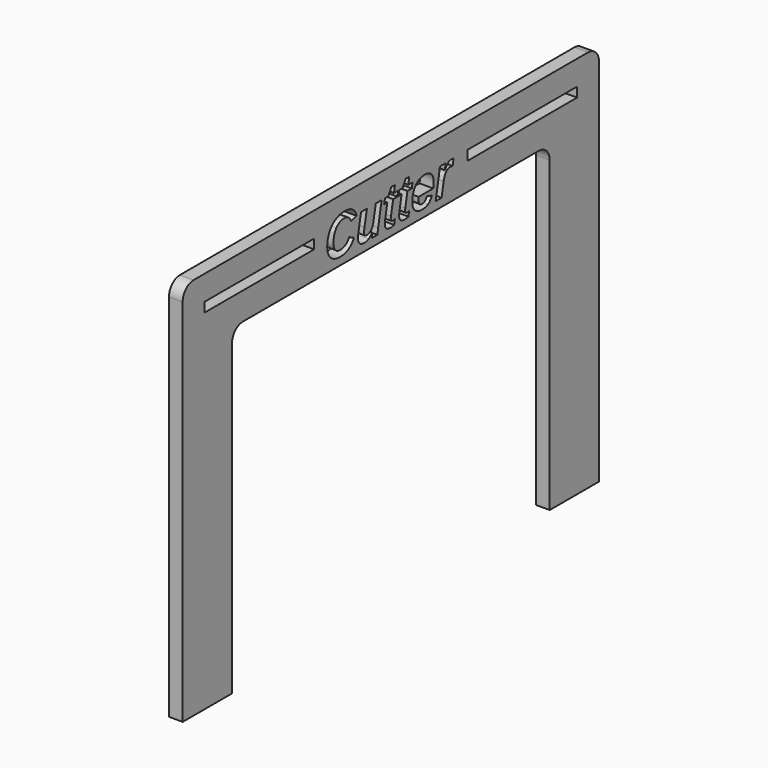
from build123d import *

# Parameters (mm, degrees)
F0_W     = 63.5
F0_H     = 4.4112131
F0_H_2   = 4.4905743218
F0_W_2   = 28.575
F0_H_3   = 149.225
F1_DEPTH = 6.35
F2_R     = 6.35


with BuildPart() as f1:
    # F0 (on Right) → F1 (new body)
    with BuildSketch(Plane.YZ):
        Polygon((-136.4888010454, 79.3362986231), (-136.4888010454, 50.7612986231), (-107.9138010454, 50.7612986231), (76.2361989546, 50.7612986231), (104.8111989546, 50.7612986231), (104.8111989546, 79.3362986231), align=None)
        with Locations((-92.0388010454, 65.6669051731)):
            Rectangle(F0_W, F0_H, mode=Mode.SUBTRACT)
        with BuildLine():
            add(Edge.make_bspline(
                [(-47.3880220701, 67.0227738236), (-49.0617207982, 64.9793044462), (-49.0617207982, 61.4645371172)],
                knots=[0, 0, 0, 1, 1, 1], degree=2))
            add(Edge.make_bspline(
                [(-49.0617207982, 61.4645371172), (-49.0617207982, 59.3587905779), (-48.0205244964, 58.2086092427)],
                knots=[0, 0, 0, 1, 1, 1], degree=2))
            add(Edge.make_bspline(
                [(-48.0205244964, 58.2086092427), (-46.9793281946, 57.0584279074), (-45.0487361733, 57.0584279074)],
                knots=[0, 0, 0, 1, 1, 1], degree=2))
            add(Edge.make_bspline(
                [(-45.0487361733, 57.0584279074), (-41.8103237506, 57.0584279074), (-39.9614705044, 60.1995322646)],
                knots=[0, 0, 0, 1, 1, 1], degree=2))
            Line((-39.9614705044, 60.1995322646), (-37.2018137644, 58.7749421844))
            add(Edge.make_bspline(
                [(-37.2018137644, 58.7749421844), (-39.7551774054, 54.2481709733), (-45.290060176, 54.2481709733)],
                knots=[0, 0, 0, 1, 1, 1], degree=2))
            add(Edge.make_bspline(
                [(-45.290060176, 54.2481709733), (-47.6137767822, 54.2481709733), (-49.2991524782, 55.1258897249)],
                knots=[0, 0, 0, 1, 1, 1], degree=2))
            add(Edge.make_bspline(
                [(-49.2991524782, 55.1258897249), (-50.9845281742, 56.0036084765), (-51.8525161192, 57.6267070105)],
                knots=[0, 0, 0, 1, 1, 1], degree=2))
            add(Edge.make_bspline(
                [(-51.8525161192, 57.6267070105), (-52.7205040642, 59.2498055445), (-52.7205040642, 61.4139369231)],
                knots=[0, 0, 0, 1, 1, 1], degree=2))
            add(Edge.make_bspline(
                [(-52.7205040642, 61.4139369231), (-52.7205040642, 64.4810871504), (-51.4438222437, 66.894327177)],
                knots=[0, 0, 0, 1, 1, 1], degree=2))
            add(Edge.make_bspline(
                [(-51.4438222437, 66.894327177), (-50.1671404232, 69.3075672035), (-47.874562398, 70.5978721532)],
                knots=[0, 0, 0, 1, 1, 1], degree=2))
            add(Edge.make_bspline(
                [(-47.874562398, 70.5978721532), (-45.5819843728, 71.8881771029), (-42.6627424051, 71.8881771029)],
                knots=[0, 0, 0, 1, 1, 1], degree=2))
            add(Edge.make_bspline(
                [(-42.6627424051, 71.8881771029), (-39.8641624389, 71.8881771029), (-38.0698017094, 70.6893417349)],
                knots=[0, 0, 0, 1, 1, 1], degree=2))
            add(Edge.make_bspline(
                [(-38.0698017094, 70.6893417349), (-36.27544098, 69.4905063669), (-35.6565616829, 67.1200818892)],
                knots=[0, 0, 0, 1, 1, 1], degree=2))
            Line((-35.6565616829, 67.1200818892), (-38.9883898486, 66.2559862667))
            add(Edge.make_bspline(
                [(-38.9883898486, 66.2559862667), (-39.3425912073, 67.556022023), (-40.3390257989, 68.3111326119)],
                knots=[0, 0, 0, 1, 1, 1], degree=2))
            add(Edge.make_bspline(
                [(-40.3390257989, 68.3111326119), (-41.3354603905, 69.0662432009), (-42.7717274386, 69.0662432009)],
                knots=[0, 0, 0, 1, 1, 1], degree=2))
            add(Edge.make_bspline(
                [(-42.7717274386, 69.0662432009), (-45.714323342, 69.0662432009), (-47.3880220701, 67.0227738236)],
                knots=[0, 0, 0, 1, 1, 1], degree=2))
        make_face(mode=Mode.SUBTRACT)
        with BuildLine():
            Line((-33.1148750097, 67.6533300886), (-29.7207696821, 67.6533300886))
            Line((-29.7207696821, 67.6533300886), (-31.1570367301, 60.4175023315))
            add(Edge.make_bspline(
                [(-31.1570367301, 60.4175023315), (-31.4723148626, 58.9228504441), (-31.4723148626, 58.4090638578)],
                knots=[0, 0, 0, 1, 1, 1], degree=2))
            add(Edge.make_bspline(
                [(-31.4723148626, 58.4090638578), (-31.4723148626, 56.8404578405), (-29.6234616165, 56.8404578405)],
                knots=[0, 0, 0, 1, 1, 1], degree=2))
            add(Edge.make_bspline(
                [(-29.6234616165, 56.8404578405), (-28.3934876674, 56.8404578405), (-27.354237527, 57.8252154643)],
                knots=[0, 0, 0, 1, 1, 1], degree=2))
            add(Edge.make_bspline(
                [(-27.354237527, 57.8252154643), (-26.3149873865, 58.809973088), (-26.0347401576, 60.2851633623)],
                knots=[0, 0, 0, 1, 1, 1], degree=2))
            Line((-26.0347401576, 60.2851633623), (-24.5984731095, 67.6533300886))
            Line((-24.5984731095, 67.6533300886), (-21.1693368783, 67.6533300886))
            Line((-21.1693368783, 67.6533300886), (-23.1894523198, 57.3036442327))
            add(Edge.make_bspline(
                [(-23.1894523198, 57.3036442327), (-23.384068451, 56.3422405447), (-23.652638712, 54.4933872986)],
                knots=[0, 0, 0, 1, 1, 1], degree=2))
            Line((-23.652638712, 54.4933872986), (-26.9105127479, 54.4933872986))
            add(Edge.make_bspline(
                [(-26.9105127479, 54.4933872986), (-26.9105127479, 54.602372332), (-26.7956892305, 55.5151219872)],
                knots=[0, 0, 0, 1, 1, 1], degree=2))
            add(Edge.make_bspline(
                [(-26.7956892305, 55.5151219872), (-26.6808657131, 56.4278716424), (-26.6185885511, 56.7431497749)],
                knots=[0, 0, 0, 1, 1, 1], degree=2))
            Line((-26.6185885511, 56.7431497749), (-26.6536194547, 56.7431497749))
            add(Edge.make_bspline(
                [(-26.6536194547, 56.7431497749), (-27.5799922391, 55.4431140187), (-28.6815195416, 54.8534271412)],
                knots=[0, 0, 0, 1, 1, 1], degree=2))
            add(Edge.make_bspline(
                [(-28.6815195416, 54.8534271412), (-29.783046844, 54.2637402638), (-31.1920676337, 54.2637402638)],
                knots=[0, 0, 0, 1, 1, 1], degree=2))
            add(Edge.make_bspline(
                [(-31.1920676337, 54.2637402638), (-33.0409208799, 54.2637402638), (-33.9770244708, 55.1511898219)],
                knots=[0, 0, 0, 1, 1, 1], degree=2))
            add(Edge.make_bspline(
                [(-33.9770244708, 55.1511898219), (-34.9131280618, 56.0386393801), (-34.9131280618, 57.7162304308)],
                knots=[0, 0, 0, 1, 1, 1], degree=2))
            add(Edge.make_bspline(
                [(-34.9131280618, 57.7162304308), (-34.9131280618, 58.0198315954), (-34.8294431254, 58.6951495706)],
                knots=[0, 0, 0, 1, 1, 1], degree=2))
            add(Edge.make_bspline(
                [(-34.8294431254, 58.6951495706), (-34.745758189, 59.3704675458), (-34.6601270913, 59.7129919367)],
                knots=[0, 0, 0, 1, 1, 1], degree=2))
            Line((-34.6601270913, 59.7129919367), (-33.1148750097, 67.6533300886))
        make_face(mode=Mode.SUBTRACT)
        with BuildLine():
            add(Edge.make_bspline(
                [(-13.9218321533, 54.5906953641), (-14.9065897771, 54.2987711674), (-16.1599176618, 54.2987711674)],
                knots=[0, 0, 0, 1, 1, 1], degree=2))
            add(Edge.make_bspline(
                [(-16.1599176618, 54.2987711674), (-17.6662465171, 54.2987711674), (-18.4933650746, 55.0110662075)],
                knots=[0, 0, 0, 1, 1, 1], degree=2))
            add(Edge.make_bspline(
                [(-18.4933650746, 55.0110662075), (-19.3204836321, 55.7233612476), (-19.3204836321, 57.0350739717)],
                knots=[0, 0, 0, 1, 1, 1], degree=2))
            add(Edge.make_bspline(
                [(-19.3204836321, 57.0350739717), (-19.3204836321, 57.8991695941), (-19.1258675009, 58.9462043798)],
                knots=[0, 0, 0, 1, 1, 1], degree=2))
            Line((-19.1258675009, 58.9462043798), (-17.8881089067, 65.3451827728))
            Line((-17.8881089067, 65.3451827728), (-19.6863619587, 65.3451827728))
            Line((-19.6863619587, 65.3451827728), (-19.238744857, 67.6533300886))
            Line((-19.238744857, 67.6533300886), (-17.2653372869, 67.6533300886))
            Line((-17.2653372869, 67.6533300886), (-15.599423204, 70.7438342516))
            Line((-15.599423204, 70.7438342516), (-13.4586457611, 70.7438342516))
            Line((-13.4586457611, 70.7438342516), (-14.0424941546, 67.6533300886))
            Line((-14.0424941546, 67.6533300886), (-11.5864385792, 67.6533300886))
            Line((-11.5864385792, 67.6533300886), (-12.0107017452, 65.3451827728))
            Line((-12.0107017452, 65.3451827728), (-14.5056805468, 65.3451827728))
            Line((-14.5056805468, 65.3451827728), (-15.7706853995, 58.8372193464))
            add(Edge.make_bspline(
                [(-15.7706853995, 58.8372193464), (-15.9030243687, 58.1560628873), (-15.9030243687, 57.755153657)],
                knots=[0, 0, 0, 1, 1, 1], degree=2))
            add(Edge.make_bspline(
                [(-15.9030243687, 57.755153657), (-15.9030243687, 57.1946591993), (-15.6169386558, 56.9202504543)],
                knots=[0, 0, 0, 1, 1, 1], degree=2))
            add(Edge.make_bspline(
                [(-15.6169386558, 56.9202504543), (-15.330852943, 56.6458417093), (-14.8443126151, 56.6458417093)],
                knots=[0, 0, 0, 1, 1, 1], degree=2))
            add(Edge.make_bspline(
                [(-14.8443126151, 56.6458417093), (-14.4550803527, 56.6458417093), (-13.532599891, 56.8054269369)],
                knots=[0, 0, 0, 1, 1, 1], degree=2))
            Line((-13.532599891, 56.8054269369), (-13.9218321533, 54.5906953641))
        make_face(mode=Mode.SUBTRACT)
        with BuildLine():
            add(Edge.make_bspline(
                [(-5.6272926427, 54.5906953641), (-6.6120502664, 54.2987711674), (-7.8653781512, 54.2987711674)],
                knots=[0, 0, 0, 1, 1, 1], degree=2))
            add(Edge.make_bspline(
                [(-7.8653781512, 54.2987711674), (-9.3717070065, 54.2987711674), (-10.198825564, 55.0110662075)],
                knots=[0, 0, 0, 1, 1, 1], degree=2))
            add(Edge.make_bspline(
                [(-10.198825564, 55.0110662075), (-11.0259441214, 55.7233612476), (-11.0259441214, 57.0350739717)],
                knots=[0, 0, 0, 1, 1, 1], degree=2))
            add(Edge.make_bspline(
                [(-11.0259441214, 57.0350739717), (-11.0259441214, 57.8991695941), (-10.8313279903, 58.9462043798)],
                knots=[0, 0, 0, 1, 1, 1], degree=2))
            Line((-10.8313279903, 58.9462043798), (-9.593569396, 65.3451827728))
            Line((-9.593569396, 65.3451827728), (-11.3918224481, 65.3451827728))
            Line((-11.3918224481, 65.3451827728), (-10.9442053464, 67.6533300886))
            Line((-10.9442053464, 67.6533300886), (-8.9707977762, 67.6533300886))
            Line((-8.9707977762, 67.6533300886), (-7.3048836934, 70.7438342516))
            Line((-7.3048836934, 70.7438342516), (-5.1641062505, 70.7438342516))
            Line((-5.1641062505, 70.7438342516), (-5.747954644, 67.6533300886))
            Line((-5.747954644, 67.6533300886), (-3.2918990686, 67.6533300886))
            Line((-3.2918990686, 67.6533300886), (-3.7161622345, 65.3451827728))
            Line((-3.7161622345, 65.3451827728), (-6.2111410362, 65.3451827728))
            Line((-6.2111410362, 65.3451827728), (-7.4761458888, 58.8372193464))
            add(Edge.make_bspline(
                [(-7.4761458888, 58.8372193464), (-7.608484858, 58.1560628873), (-7.608484858, 57.755153657)],
                knots=[0, 0, 0, 1, 1, 1], degree=2))
            add(Edge.make_bspline(
                [(-7.608484858, 57.755153657), (-7.608484858, 57.1946591993), (-7.3223991452, 56.9202504543)],
                knots=[0, 0, 0, 1, 1, 1], degree=2))
            add(Edge.make_bspline(
                [(-7.3223991452, 56.9202504543), (-7.0363134324, 56.6458417093), (-6.5497731044, 56.6458417093)],
                knots=[0, 0, 0, 1, 1, 1], degree=2))
            add(Edge.make_bspline(
                [(-6.5497731044, 56.6458417093), (-6.1605408421, 56.6458417093), (-5.2380603803, 56.8054269369)],
                knots=[0, 0, 0, 1, 1, 1], degree=2))
            Line((-5.2380603803, 56.8054269369), (-5.6272926427, 54.5906953641))
        make_face(mode=Mode.SUBTRACT)
        with BuildLine():
            Line((8.7237008701, 60.2851633623), (0.2111912926, 60.2851633623))
            add(Edge.make_bspline(
                [(0.2111912926, 60.2851633623), (0.1255601948, 59.8219769701), (0.1255601948, 59.1992053504)],
                knots=[0, 0, 0, 1, 1, 1], degree=2))
            add(Edge.make_bspline(
                [(0.1255601948, 59.1992053504), (0.1255601948, 57.910846562), (0.6918931366, 57.2238516189)],
                knots=[0, 0, 0, 1, 1, 1], degree=2))
            add(Edge.make_bspline(
                [(0.6918931366, 57.2238516189), (1.2582260783, 56.5368566759), (2.3636457034, 56.5368566759)],
                knots=[0, 0, 0, 1, 1, 1], degree=2))
            add(Edge.make_bspline(
                [(2.3636457034, 56.5368566759), (4.1502217875, 56.5368566759), (4.9559325706, 58.5920030211)],
                knots=[0, 0, 0, 1, 1, 1], degree=2))
            Line((4.9559325706, 58.5920030211), (7.9335593776, 57.6928764951))
            add(Edge.make_bspline(
                [(7.9335593776, 57.6928764951), (7.0227558837, 55.7583921512), (5.6721199333, 55.0032815622)],
                knots=[0, 0, 0, 1, 1, 1], degree=2))
            add(Edge.make_bspline(
                [(5.6721199333, 55.0032815622), (4.321483983, 54.2481709733), (2.1339986686, 54.2481709733)],
                knots=[0, 0, 0, 1, 1, 1], degree=2))
            add(Edge.make_bspline(
                [(2.1339986686, 54.2481709733), (-0.4582881987, 54.2481709733), (-1.9179091825, 55.6532994404)],
                knots=[0, 0, 0, 1, 1, 1], degree=2))
            add(Edge.make_bspline(
                [(-1.9179091825, 55.6532994404), (-3.3775301663, 57.0584279074), (-3.3775301663, 59.5767606448)],
                knots=[0, 0, 0, 1, 1, 1], degree=2))
            add(Edge.make_bspline(
                [(-3.3775301663, 59.5767606448), (-3.3775301663, 62.0950933822), (-2.501757576, 63.9867621772)],
                knots=[0, 0, 0, 1, 1, 1], degree=2))
            add(Edge.make_bspline(
                [(-2.501757576, 63.9867621772), (-1.6259849857, 65.8784309723), (-0.0145634196, 66.8884886931)],
                knots=[0, 0, 0, 1, 1, 1], degree=2))
            add(Edge.make_bspline(
                [(-0.0145634196, 66.8884886931), (1.5968581465, 67.8985464138), (3.7142816537, 67.8985464138)],
                knots=[0, 0, 0, 1, 1, 1], degree=2))
            add(Edge.make_bspline(
                [(3.7142816537, 67.8985464138), (6.2559683268, 67.8985464138), (7.6357966969, 66.5907260124)],
                knots=[0, 0, 0, 1, 1, 1], degree=2))
            add(Edge.make_bspline(
                [(7.6357966969, 66.5907260124), (9.0156250669, 65.2829056109), (9.0156250669, 62.8969118427)],
                knots=[0, 0, 0, 1, 1, 1], degree=2))
            add(Edge.make_bspline(
                [(9.0156250669, 62.8969118427), (9.0156250669, 61.694184152), (8.7237008701, 60.2851633623)],
                knots=[0, 0, 0, 1, 1, 1], degree=2))
        make_face(mode=Mode.SUBTRACT)
        with BuildLine():
            Line((20.5330077098, 67.7272842184), (19.9764055746, 64.8703194128))
            add(Edge.make_bspline(
                [(19.9764055746, 64.8703194128), (19.135663888, 65.0532585761), (18.586846398, 65.0532585761)],
                knots=[0, 0, 0, 1, 1, 1], degree=2))
            add(Edge.make_bspline(
                [(18.586846398, 65.0532585761), (17.0921945106, 65.0532585761), (16.1502524357, 63.9945468225)],
                knots=[0, 0, 0, 1, 1, 1], degree=2))
            add(Edge.make_bspline(
                [(16.1502524357, 63.9945468225), (15.2083103609, 62.9358350689), (14.7801548723, 60.7444574319)],
                knots=[0, 0, 0, 1, 1, 1], degree=2))
            Line((14.7801548723, 60.7444574319), (13.5540732459, 54.4933872986))
            Line((13.5540732459, 54.4933872986), (10.1327216598, 54.4933872986))
            Line((10.1327216598, 54.4933872986), (12.0944522621, 64.5900721839))
            add(Edge.make_bspline(
                [(12.0944522621, 64.5900721839), (12.3863764588, 66.0496931677), (12.6043465257, 67.6533300886)],
                knots=[0, 0, 0, 1, 1, 1], degree=2))
            Line((12.6043465257, 67.6533300886), (15.8622205616, 67.6533300886))
            Line((15.8622205616, 67.6533300886), (15.5975426232, 65.5631528398))
            Line((15.5975426232, 65.5631528398), (15.5002345576, 64.9676274784))
            Line((15.5002345576, 64.9676274784), (15.5469424291, 64.9676274784))
            add(Edge.make_bspline(
                [(15.5469424291, 64.9676274784), (16.4343919873, 66.594618335), (17.2984876097, 67.2465823744)],
                knots=[0, 0, 0, 1, 1, 1], degree=2))
            add(Edge.make_bspline(
                [(17.2984876097, 67.2465823744), (18.1625832321, 67.8985464138), (19.279679825, 67.8985464138)],
                knots=[0, 0, 0, 1, 1, 1], degree=2))
            add(Edge.make_bspline(
                [(19.279679825, 67.8985464138), (19.8518512507, 67.8985464138), (20.5330077098, 67.7272842184)],
                knots=[0, 0, 0, 1, 1, 1], degree=2))
        make_face(mode=Mode.SUBTRACT)
        with Locations((60.3611989546, 65.706585784)):
            Rectangle(F0_W, F0_H_2, mode=Mode.SUBTRACT)
        with Locations((-122.2013010454, -23.8512013769)):
            Rectangle(F0_W_2, F0_H_3)
        with Locations((90.5236989546, -23.8512013769)):
            Rectangle(F0_W_2, F0_H_3)
    extrude(amount=F1_DEPTH)

    # F2
    f2_edges = [f1.edges().sort_by_distance(p)[0] for p in [
        (3.175, -136.488801, 79.336299),
        (3.175, 104.811199, 79.336299),
        (3.175, -107.913801, 50.761299),
        (3.175, 76.236199, 50.761299),
    ]]
    fillet(f2_edges, radius=F2_R)


solid = f1.part
